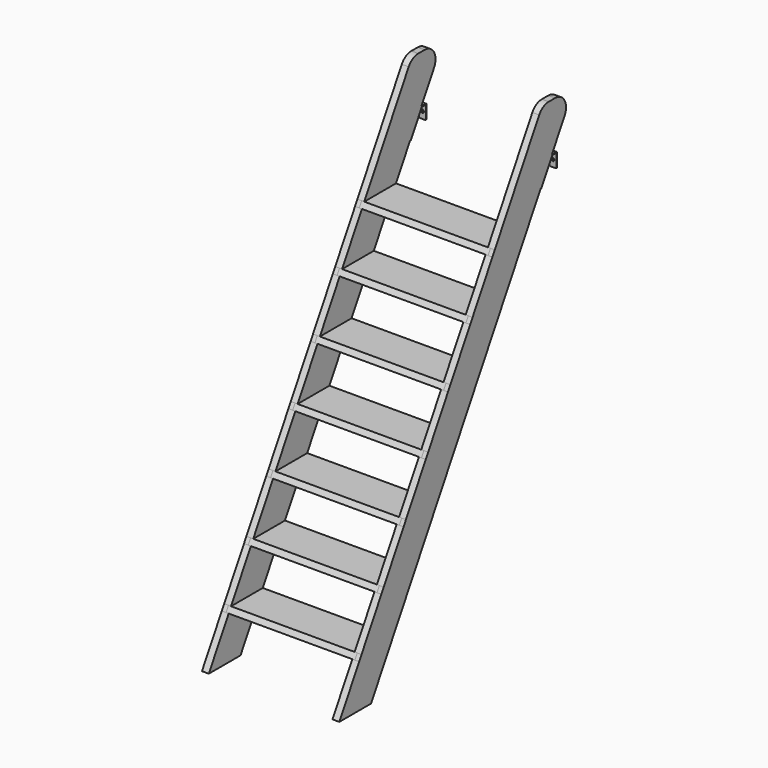
from build123d import *

# Parameters (mm, degrees)
F1_DEPTH       = 25.4
F2_DEPTH       = 9.525
F3_DEPTH       = 25.4
F6_DEPTH       = 476.25
F8_D           = 4.4958
F8_CSINK_D     = 9.1186
F8_CSINK_ANGLE = 82
F11_D          = 10.0838
F11_DEPTH      = 6.35
F11_START      = 20.715374
F11_TIP        = 3.029479
F12_R          = 3.175


# Not quite as in the source:
# - a feature names something its author has since deleted; it is built from what else it names


with BuildPart() as f1:
    # F0 (on Right) → F1 (new body)
    with BuildSketch(Plane.YZ):
        with BuildLine():
            ThreePointArc((-43.994091, -76.2), (-43.994091, -25.4), (-87.988181, 0))
            Line((-87.988181, 0), (-117.317575, 0))
            ThreePointArc((-117.317575, 0), (-142.717575, -6.805909), (-161.311665, -25.4))
            Line((-161.311665, -25.4), (-366.617421, -381))
            Line((-366.617421, -381), (-219.970453, -381))
            Line((-219.970453, -381), (-154.369421, -267.375681))
            Line((-154.369421, -267.375681), (-102.652878, -177.8))
            Line((-102.652878, -177.8), (-43.994091, -76.2))
        make_face()
        Polygon((-219.970453, -381), (-366.617421, -381), (-377.615944, -400.05), (-230.968975, -400.05), align=None)
        Polygon((-230.968975, -400.05), (-377.615944, -400.05), (-469.270299, -558.8), (-322.62333, -558.8), align=None)
        Polygon((-322.62333, -558.8), (-469.270299, -558.8), (-480.268821, -577.85), (-333.621853, -577.85), align=None)
        Polygon((-333.621853, -577.85), (-480.268821, -577.85), (-571.923177, -736.6), (-425.276208, -736.6), align=None)
        Polygon((-425.276208, -736.6), (-571.923177, -736.6), (-582.921699, -755.65), (-436.274731, -755.65), align=None)
        Polygon((-436.274731, -755.65), (-582.921699, -755.65), (-674.576055, -914.4), (-527.929086, -914.4), align=None)
        Polygon((-538.927609, -933.45), (-685.574577, -933.45), (-777.228932, -1092.2), (-630.581964, -1092.2), align=None)
        Polygon((-641.580487, -1111.25), (-788.227455, -1111.25), (-879.88181, -1270), (-733.234842, -1270), align=None)
        Polygon((-744.233364, -1289.05), (-890.880333, -1289.05), (-982.534688, -1447.8), (-835.88772, -1447.8), align=None)
        Polygon((-846.886242, -1466.85), (-993.533211, -1466.85), (-1085.187566, -1625.6), (-938.540598, -1625.6), align=None)
        Polygon((-835.88772, -1447.8), (-982.534688, -1447.8), (-993.533211, -1466.85), (-846.886242, -1466.85), align=None)
        Polygon((-733.234842, -1270), (-879.88181, -1270), (-890.880333, -1289.05), (-744.233364, -1289.05), align=None)
        Polygon((-630.581964, -1092.2), (-777.228932, -1092.2), (-788.227455, -1111.25), (-641.580487, -1111.25), align=None)
        Polygon((-527.929086, -914.4), (-674.576055, -914.4), (-685.574577, -933.45), (-538.927609, -933.45), align=None)
    extrude(amount=F1_DEPTH)

    # F0 (on Right) → F2 (cut)
    with BuildSketch(Plane.YZ):
        Polygon((-219.970453, -381), (-366.617421, -381), (-377.615944, -400.05), (-230.968975, -400.05), align=None)
        Polygon((-322.62333, -558.8), (-469.270299, -558.8), (-480.268821, -577.85), (-333.621853, -577.85), align=None)
        Polygon((-425.276208, -736.6), (-571.923177, -736.6), (-582.921699, -755.65), (-436.274731, -755.65), align=None)
        Polygon((-527.929086, -914.4), (-674.576055, -914.4), (-685.574577, -933.45), (-538.927609, -933.45), align=None)
        Polygon((-630.581964, -1092.2), (-777.228932, -1092.2), (-788.227455, -1111.25), (-641.580487, -1111.25), align=None)
        Polygon((-733.234842, -1270), (-879.88181, -1270), (-890.880333, -1289.05), (-744.233364, -1289.05), align=None)
        Polygon((-835.88772, -1447.8), (-982.534688, -1447.8), (-993.533211, -1466.85), (-846.886242, -1466.85), align=None)
    extrude(amount=F2_DEPTH, mode=Mode.SUBTRACT)


with BuildPart() as f3:
    # F0 (on Right) → F3 (new body)
    with BuildSketch(Plane.YZ):
        with BuildLine():
            Line((-81.769791, -177.8), (-102.652878, -177.8))
            Line((-102.652878, -177.8), (-154.369421, -267.375681))
            Line((-154.369421, -267.375681), (-151.619791, -268.963181))
            Line((-151.619791, -268.963181), (-100.819791, -180.975))
            Line((-100.819791, -180.975), (-84.944791, -180.975))
            ThreePointArc((-84.944791, -180.975), (-82.699727, -181.904936), (-81.769791, -184.15))
            Line((-81.769791, -184.15), (-81.769791, -231.775))
            Line((-81.769791, -231.775), (-78.594791, -231.775))
            Line((-78.594791, -231.775), (-78.594791, -180.975))
            ThreePointArc((-78.594791, -180.975), (-79.524727, -178.729936), (-81.769791, -177.8))
        make_face()
    extrude(amount=F3_DEPTH)

    # F8 (through all)
    with Locations(Plane(origin=(0, 2.749631, -1.5875), x_dir=(-1, 0, 0), z_dir=(0, 0.866025, -0.5))):
        with Locations((-12.7, -219.838843), (-12.7, -289.688843)):
            CounterSinkHole(F8_D / 2, F8_CSINK_D / 2, counter_sink_angle=F8_CSINK_ANGLE)

    # F11
    # its depths count from where the whole tool has entered the part; down to there all is cleared
    with Locations(Plane(origin=(0, 46.743721, -26.9875), x_dir=(-1, 0, 0), z_dir=(0, 0.866025, -0.5))):
        with Locations((-12.7, -219.838843)):
            Hole(F11_D / 2, depth=F11_START)
    with Locations(Plane(origin=(0, 46.743721, -26.9875), x_dir=(-1, 0, 0), z_dir=(0, 0.866025, -0.5)).offset(-F11_START)):
        with Locations((-12.7, -219.838843)):
            Hole(F11_D / 2, depth=F11_DEPTH)
            with Locations((0, 0, -(F11_DEPTH + F11_TIP / 2))):  # 118° drill point
                Cone(0, F11_D / 2, F11_TIP, mode=Mode.SUBTRACT)

    # F12
    f12_edges = [f3.edges().sort_by_distance(p)[0] for p in [
        (25.4, -80.182291, -231.775),
        (0, -80.182291, -231.775),
    ]]
    fillet(f12_edges, radius=F12_R)


with BuildPart() as f5_1:
    # F5: instance of F1
    add(f1.part.mirror(Plane.YZ.offset(-228.6)))


with BuildPart() as f6:
    # F6 (new, through all): a face of the model
    f6_faces = [f1.part.faces().sort_by_distance(p)[0] for p in [
        (9.525, -298.793198, -390.525),
    ]]
    extrude(f6_faces, amount=F6_DEPTH)


with BuildPart() as f6b:
    # F6#2 (new, through all): a face of the model
    f6_2_faces = [f1.part.faces().sort_by_distance(p)[0] for p in [
        (9.525, -401.446076, -568.325),
    ]]
    extrude(f6_2_faces, amount=F6_DEPTH)


with BuildPart() as f6c:
    # F6#3 (new, through all): a face of the model
    f6_3_faces = [f1.part.faces().sort_by_distance(p)[0] for p in [
        (9.525, -504.098954, -746.125),
    ]]
    extrude(f6_3_faces, amount=F6_DEPTH)


with BuildPart() as f6d:
    # F6#4 (new, through all): a face of the model
    f6_4_faces = [f1.part.faces().sort_by_distance(p)[0] for p in [
        (9.525, -606.751832, -923.925),
    ]]
    extrude(f6_4_faces, amount=F6_DEPTH)


with BuildPart() as f6e:
    # F6#5 (new, through all): a face of the model
    f6_5_faces = [f1.part.faces().sort_by_distance(p)[0] for p in [
        (9.525, -709.40471, -1101.725),
    ]]
    extrude(f6_5_faces, amount=F6_DEPTH)


with BuildPart() as f6f:
    # F6#6 (new, through all): a face of the model
    f6_6_faces = [f1.part.faces().sort_by_distance(p)[0] for p in [
        (9.525, -812.057587, -1279.525),
    ]]
    extrude(f6_6_faces, amount=F6_DEPTH)


with BuildPart() as f6g:
    # F6#7 (new, through all): a face of the model
    f6_7_faces = [f1.part.faces().sort_by_distance(p)[0] for p in [
        (9.525, -914.710465, -1457.325),
    ]]
    extrude(f6_7_faces, amount=F6_DEPTH)


with BuildPart() as f13_1:
    # F13: instance of F3
    add(f3.part.mirror(Plane.YZ.offset(-228.6)))


solid = Compound([f1.part, f3.part, f5_1.part, f6.part, f6b.part, f6c.part, f6d.part, f6e.part, f6f.part, f6g.part, f13_1.part])
